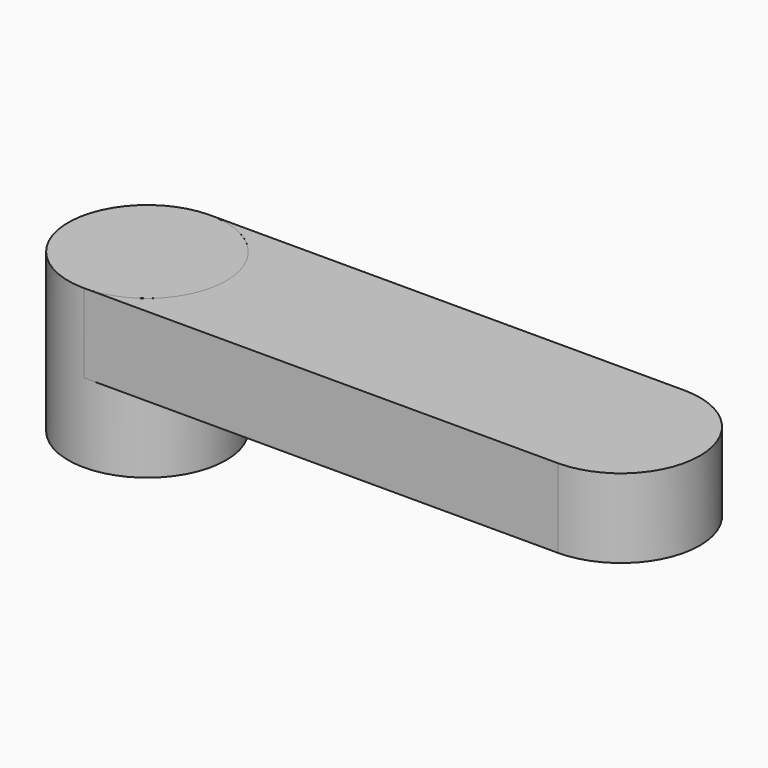
from build123d import *

# Parameters (mm, degrees)
F0_R     = 5
F2_DEPTH = 5
F3_DEPTH = 5


with BuildPart() as f2:
    # F0 (on Top) → F2 (new body)
    with BuildSketch(Plane.XY):
        Circle(F0_R)
    extrude(amount=F2_DEPTH)

    # F3 (add): a face of the model
    f3_faces = [f2.faces().sort_by_distance(p)[0] for p in [
        (0, 0, 0),
    ]]
    extrude(f3_faces, amount=F3_DEPTH)


with BuildPart() as f2b:
    # F1 (on Top) → F2, piece 2 (new body)
    with BuildSketch(Plane.XY):
        with BuildLine():
            Line((30, 5), (0, 5))
            ThreePointArc((0, 5), (5, 0), (0, -5))
            Line((0, -5), (30, -5))
            ThreePointArc((30, -5), (35, 0), (30, 5))
        make_face()
    extrude(amount=F2_DEPTH)


solid = Compound([f2.part, f2b.part])
